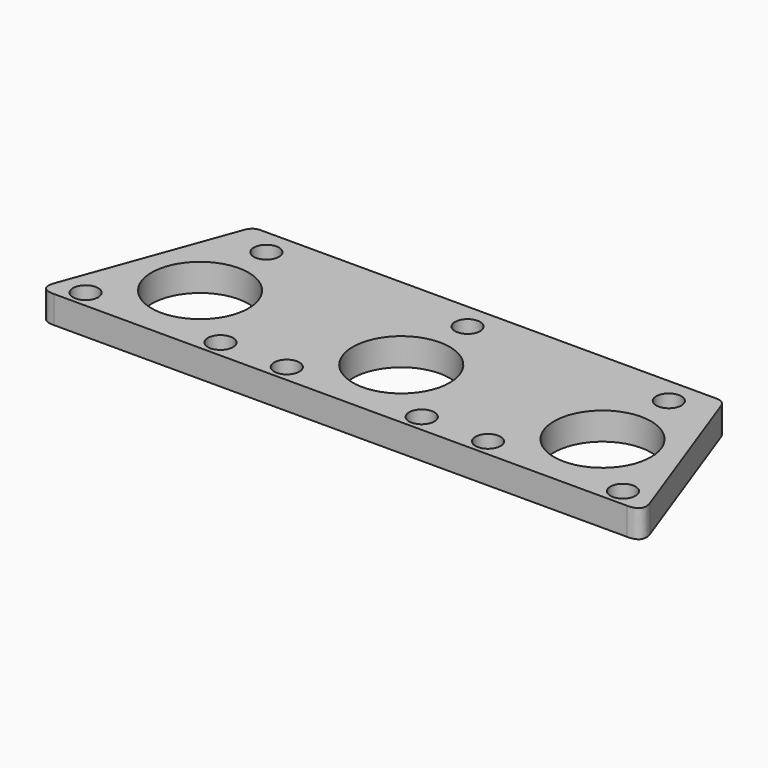
from build123d import *

# Parameters (mm, degrees)
F0_R        = 5.5
F0_R_2      = 21.2
F1_DEPTH    = 6
F2_T1_DEPTH = 47.7037001686
F2_T3_DEPTH = 29.5051884552


# Not quite as in the source:
# - a fillet or chamfer that OpenCascade refuses, or shapes differently, is made with other operations: its cross-section is extruded or revolved along the edge and cut away or added


with BuildPart() as f1:
    # F0 (on Top) → F1 (new body, symmetric)
    with BuildSketch(Plane.XY):
        Polygon((103.0366095362, 47.75), (-103.0366095362, 47.75), (-132.5, -33.2), (0, -33.2), (132.5, -33.2), align=None)
        with Locations((-117.5, -25.7)):
            Circle(F0_R, mode=Mode.SUBTRACT)
        with Locations((-58.5, -25.7)):
            Circle(F0_R, mode=Mode.SUBTRACT)
        with Locations((-29.5, -25.7)):
            Circle(F0_R, mode=Mode.SUBTRACT)
        with Locations((-88, 0)):
            Circle(F0_R_2, mode=Mode.SUBTRACT)
        with Locations((29.5, -25.7)):
            Circle(F0_R, mode=Mode.SUBTRACT)
        with Locations((58.5, -25.7)):
            Circle(F0_R, mode=Mode.SUBTRACT)
        with Locations((117.5, -25.7)):
            Circle(F0_R, mode=Mode.SUBTRACT)
        Circle(F0_R_2, mode=Mode.SUBTRACT)
        with Locations((88, 0)):
            Circle(F0_R_2, mode=Mode.SUBTRACT)
        with Locations((-88, 36.25)):
            Circle(F0_R, mode=Mode.SUBTRACT)
        with Locations((0, 36.25)):
            Circle(F0_R, mode=Mode.SUBTRACT)
        with Locations((88, 36.25)):
            Circle(F0_R, mode=Mode.SUBTRACT)
    extrude(amount=F1_DEPTH, both=True)

    # F2: fillet of radius 5 on 4 edges, made by hand

    # F2_s2 → F2_t1 (cut)
    with BuildSketch(Plane.XY.offset(-23.8518500843)):
        with BuildLine():
            add(Edge.make_bspline(
                [(-125.3592599663, -33.2), (-132.5, -33.2), (-130.0577230702, -26.4898992834)],
                knots=[0, 0, 0, 1, 1, 1], degree=2, weights=[1, 1, 1]))
            Line((-130.0577230702, -26.4898992834), (-132.5, -33.2))
            Line((-132.5, -33.2), (-125.3592599663, -33.2))
        make_face()
        with BuildLine():
            add(Edge.make_bspline(
                [(130.0577230702, -26.4898992834), (132.5, -33.2), (125.3592599663, -33.2)],
                knots=[0, 0, 0, 1, 1, 1], degree=2, weights=[1, 1, 1]))
            Line((125.3592599663, -33.2), (132.5, -33.2))
            Line((132.5, -33.2), (130.0577230702, -26.4898992834))
        make_face()
    extrude(amount=F2_T1_DEPTH, mode=Mode.SUBTRACT)

    # F2_s4 → F2_t3 (cut)
    with BuildSketch(Plane.XY.offset(-14.7525942276)):
        with BuildLine():
            add(Edge.make_bspline(
                [(-99.5355718451, 47.75), (-103.0366095362, 47.75), (-104.234034949, 44.4601007166)],
                knots=[0, 0, 0, 1, 1, 1], degree=2, weights=[1, 1, 1]))
            Line((-104.234034949, 44.4601007166), (-103.0366095362, 47.75))
            Line((-103.0366095362, 47.75), (-99.5355718451, 47.75))
        make_face()
        with BuildLine():
            add(Edge.make_bspline(
                [(99.5355718451, 47.75), (103.0366095362, 47.75), (104.234034949, 44.4601007166)],
                knots=[0, 0, 0, 1, 1, 1], degree=2, weights=[1, 1, 1]))
            Line((104.234034949, 44.4601007166), (103.0366095362, 47.75))
            Line((103.0366095362, 47.75), (99.5355718451, 47.75))
        make_face()
    extrude(amount=F2_T3_DEPTH, mode=Mode.SUBTRACT)


solid = f1.part
